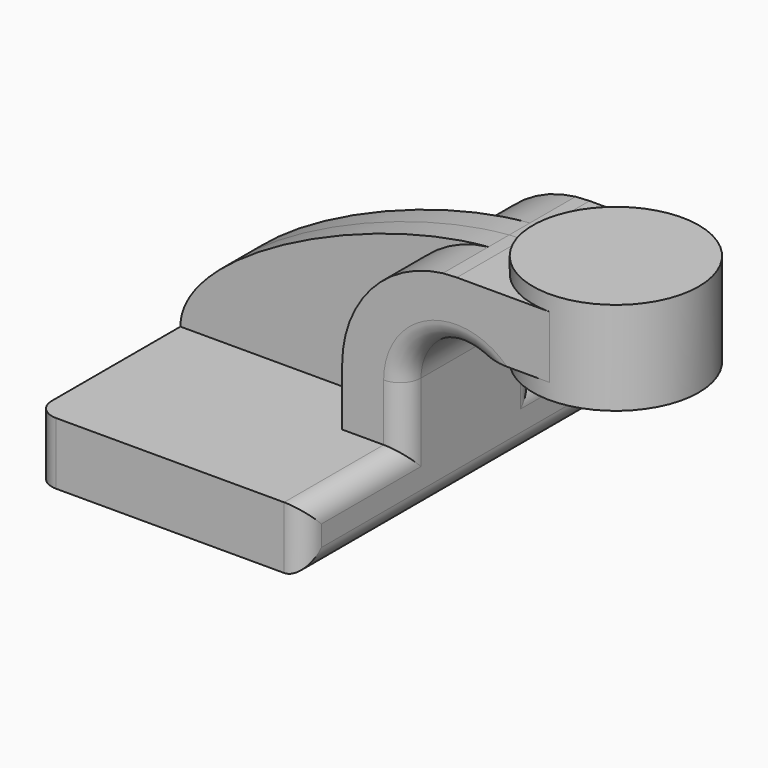
from build123d import *

# Parameters (mm, degrees)
F1_DEPTH     = 63.5
F0_W         = 25.4
F0_H         = 19.05
F2_DEPTH     = 25.4
F3_DEPTH     = 7.9375
F5_T1_DEPTH  = 50.8
F5_T3_DEPTH  = 158.75
F5_T5_DEPTH  = 53.975
F5_T7_DEPTH  = 17.4757259071
F5_T9_DEPTH  = 53.975
F5_T12_ANGLE = 147.7854112401
F5_T14_ANGLE = 147.7854112401
F5_T19_DEPTH = 53.975
F5_T23_DEPTH = 33.3507259071
F5_T30_DEPTH = 33.3507259071
F5_T34_DEPTH = 53.975


# Not quite as in the source:
# - a fillet or chamfer that OpenCascade refuses, or shapes differently, is made with other operations: its cross-section is extruded or revolved along the edge and cut away or added


with BuildPart() as f1:
    # F0 (on Front) → F1 (new body, symmetric)
    with BuildSketch(Plane.XZ):
        Polygon((-41.275, -9.525), (41.275, -9.525), (41.275, 9.525), (22.225, 9.525), (-41.275, 9.525), align=None)
    extrude(amount=F1_DEPTH, both=True)

    # F0 (on Front) → F2 (join, symmetric)
    with BuildSketch(Plane.XZ):
        with BuildLine():
            Line((22.225, 9.525), (41.275, 9.525))
            Line((41.275, 9.525), (41.275, 27.0007259071))
            ThreePointArc((41.275, 27.0007259071), (45.9704586348, 38.2716389076), (57.2792179355, 42.8752))
            Line((57.2792179355, 42.8752), (60.325, 42.8752))
            Line((60.325, 42.8752), (60.325, 61.9252))
            Line((60.325, 61.9252), (57.3416620374, 61.9252))
            add(Edge.make_bspline(
                [(53.0544398296, 61.6847569862), (54.513344238, 61.8019382233), (55.9438787453, 61.882664375), (57.3416620374, 61.9252)],
                knots=[107.5126961268, 107.5126961268, 107.5126961268, 107.5126961268, 111.6737524732, 111.6737524732, 111.6737524732, 111.6737524732], degree=3))
            ThreePointArc((53.0544398296, 61.6847569862), (31.0464268351, 50.2032924252), (22.225, 27.0007259071))
            Line((22.225, 27.0007259071), (22.225, 9.525))
        make_face()
        with Locations((73.025, 52.4002)):
            Rectangle(F0_W, F0_H)
    extrude(amount=F2_DEPTH, both=True)

    # F0 (on Front) → F3 (join, symmetric)
    with BuildSketch(Plane.XZ):
        with BuildLine():
            add(Edge.make_bspline(
                [(-41.275, 9.525), (-41.275, 31.2921475952), (15.3595053514, 58.6570472681), (53.0544398296, 61.6847569862)],
                knots=[0, 0, 0, 0, 107.5126961268, 107.5126961268, 107.5126961268, 107.5126961268], degree=3))
            Line((-41.275, 9.525), (22.225, 9.525))
            Line((22.225, 9.525), (22.225, 27.0007259071))
            ThreePointArc((22.225, 27.0007259071), (31.0464268351, 50.2032924252), (53.0544398296, 61.6847569862))
        make_face()
    extrude(amount=F3_DEPTH, both=True)

    # F0 (on Front) → F4 (revolve)
    with BuildSketch(Plane.XZ):
        Polygon((85.725, 61.9252), (85.725, 42.8752), (85.725, 38.1), (111.125, 38.1), (111.125, 66.675), (85.725, 66.675), align=None)
    revolve(axis=Axis((85.725, 0, 52.3875), (0, 0, 1)))

    # F5: fillet of radius 6.35 on 12 edges, made by hand

    # F5_s2 → F5_t1 (cut)
    with BuildSketch(Plane.XY.offset(-25.4)):
        with BuildLine():
            ThreePointArc((41.275, -57.15), (39.4151280605, -61.6401280605), (34.925, -63.5))
            Line((34.925, -63.5), (41.275, -63.5))
            Line((41.275, -63.5), (41.275, -57.15))
        make_face()
        with BuildLine():
            ThreePointArc((-34.925, -63.5), (-39.4151280605, -61.6401280605), (-41.275, -57.15))
            Line((-41.275, -57.15), (-41.275, -63.5))
            Line((-41.275, -63.5), (-34.925, -63.5))
        make_face()
        with BuildLine():
            ThreePointArc((34.925, 63.5), (39.4151280605, 61.6401280605), (41.275, 57.15))
            Line((41.275, 57.15), (41.275, 63.5))
            Line((41.275, 63.5), (34.925, 63.5))
        make_face()
        with BuildLine():
            ThreePointArc((-34.925, 63.5), (-39.4151280605, 61.6401280605), (-41.275, 57.15))
            Line((-41.275, 57.15), (-41.275, 63.5))
            Line((-41.275, 63.5), (-34.925, 63.5))
        make_face()
    extrude(amount=F5_T1_DEPTH, mode=Mode.SUBTRACT)

    # F5_s4 → F5_t3 (cut)
    with BuildSketch(Plane.XZ.offset(-79.375)):
        with BuildLine():
            ThreePointArc((34.925, -9.525), (39.4151280605, -7.6651280605), (41.275, -3.175))
            Line((41.275, -3.175), (41.275, -9.525))
            Line((41.275, -9.525), (34.925, -9.525))
        make_face()
    extrude(amount=F5_T3_DEPTH, mode=Mode.SUBTRACT)

    # F5_s6 → F5_t5 (cut)
    with BuildSketch(Plane.XZ.offset(-79.375)):
        with BuildLine():
            ThreePointArc((41.275, 3.175), (39.4151280605, 7.6651280605), (34.925, 9.525))
            Line((34.925, 9.525), (41.275, 9.525))
            Line((41.275, 9.525), (41.275, 3.175))
        make_face()
    extrude(amount=F5_T5_DEPTH, mode=Mode.SUBTRACT)

    # F5_s8 → F5_t7 (cut)
    with BuildSketch(Plane.XY.offset(9.525)):
        with BuildLine():
            ThreePointArc((41.275, 19.05), (39.4151280605, 23.5401280605), (34.925, 25.4))
            Line((34.925, 25.4), (41.275, 25.4))
            Line((41.275, 25.4), (41.275, 19.05))
        make_face()
        with BuildLine():
            ThreePointArc((41.275, -19.05), (39.4151280605, -23.5401280605), (34.925, -25.4))
            Line((34.925, -25.4), (41.275, -25.4))
            Line((41.275, -25.4), (41.275, -19.05))
        make_face()
    extrude(amount=F5_T7_DEPTH, mode=Mode.SUBTRACT)

    # F5_s10 → F5_t9 (cut)
    with BuildSketch(Plane.XZ.offset(25.4)):
        with BuildLine():
            ThreePointArc((41.275, 3.175), (39.4151280605, 7.6651280605), (34.925, 9.525))
            Line((34.925, 9.525), (41.275, 9.525))
            Line((41.275, 9.525), (41.275, 3.175))
        make_face()
    extrude(amount=F5_T9_DEPTH, mode=Mode.SUBTRACT)

    # F5_s11 → F5_t12 (revolve, cut)
    with BuildSketch(Plane.XY.offset(27.0007259071)):
        with BuildLine():
            ThreePointArc((34.925, 25.4), (39.4151280605, 23.5401280605), (41.275, 19.05))
            Line((41.275, 19.05), (41.275, 25.4))
            Line((41.275, 25.4), (34.925, 25.4))
        make_face()
    revolve(axis=Axis((57.15, 25.4, 27.0007259071), (0, 1, 0)), revolution_arc=F5_T12_ANGLE, mode=Mode.SUBTRACT)

    # F5_s13 → F5_t14 (revolve, cut)
    with BuildSketch(Plane.XY.offset(27.0007259071)):
        with BuildLine():
            ThreePointArc((41.275, -19.05), (39.4151280605, -23.5401280605), (34.925, -25.4))
            Line((34.925, -25.4), (41.275, -25.4))
            Line((41.275, -25.4), (41.275, -19.05))
        make_face()
    revolve(axis=Axis((57.15, -25.4, 27.0007259071), (0, 1, 0)), revolution_arc=F5_T14_ANGLE, mode=Mode.SUBTRACT)


with BuildPart() as f5_tool17:
    # F5_s18 → F5_t19 (new body)
    with BuildSketch(Plane.XZ.offset(-63.5)):
        with BuildLine():
            ThreePointArc((41.275, 3.175), (39.4151280605, 7.6651280605), (34.925, 9.525))
            Line((34.925, 9.525), (41.275, 9.525))
            Line((41.275, 9.525), (41.275, 3.175))
        make_face()
    extrude(amount=F5_T19_DEPTH)

    split(bisect_by=Plane.XZ.offset(-25.4), keep=Keep.TOP)


with BuildPart() as f5_tool21:
    # F5_s22 → F5_t23 (new body)
    with BuildSketch(Plane.XY.offset(-6.35)):
        with BuildLine():
            ThreePointArc((41.275, 19.05), (39.4151280605, 23.5401280605), (34.925, 25.4))
            Line((34.925, 25.4), (41.275, 25.4))
            Line((41.275, 25.4), (41.275, 19.05))
        make_face()
    extrude(amount=F5_T23_DEPTH)

    split(bisect_by=Plane.XY.offset(9.525), keep=Keep.BOTTOM)


with BuildPart() as f5_tool17_1:
    add(f5_tool17.part)

    # F5_t25: intersect F5_tool21
    add(f5_tool21.part, mode=Mode.INTERSECT)


with BuildPart() as f1_1:
    add(f1.part)

    # F5_t15: cut F5_tool17
    add(f5_tool17_1.part, mode=Mode.SUBTRACT)


with BuildPart() as f5_tool28:
    # F5_s29 → F5_t30 (new body)
    with BuildSketch(Plane.XY.offset(-6.35)):
        with BuildLine():
            ThreePointArc((41.275, -19.05), (39.4151280605, -23.5401280605), (34.925, -25.4))
            Line((34.925, -25.4), (41.275, -25.4))
            Line((41.275, -25.4), (41.275, -19.05))
        make_face()
    extrude(amount=F5_T30_DEPTH)

    split(bisect_by=Plane.XY.offset(9.525), keep=Keep.BOTTOM)


with BuildPart() as f5_tool32:
    # F5_s33 → F5_t34 (new body)
    with BuildSketch(Plane.XZ.offset(9.525)):
        with BuildLine():
            ThreePointArc((41.275, 3.175), (39.4151280605, 7.6651280605), (34.925, 9.525))
            Line((34.925, 9.525), (41.275, 9.525))
            Line((41.275, 9.525), (41.275, 3.175))
        make_face()
    extrude(amount=F5_T34_DEPTH)

    split(bisect_by=Plane.XZ.offset(25.4), keep=Keep.BOTTOM)


with BuildPart() as f5_tool28_1:
    add(f5_tool28.part)

    # F5_t36: intersect F5_tool32
    add(f5_tool32.part, mode=Mode.INTERSECT)


with BuildPart() as f1_2:
    add(f1_1.part)

    # F5_t26: cut F5_tool28
    add(f5_tool28_1.part, mode=Mode.SUBTRACT)


solid = f1_2.part
